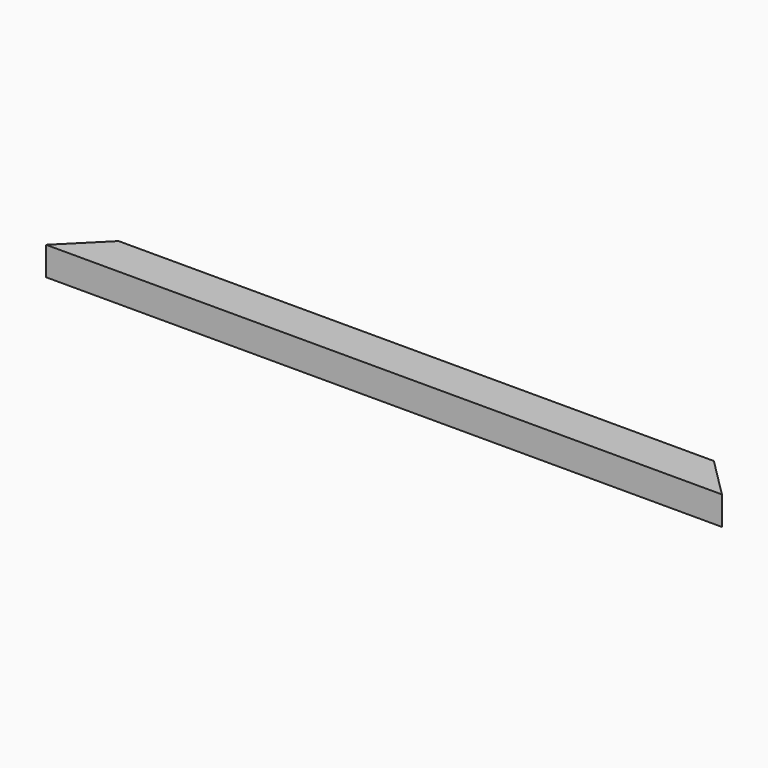
from build123d import *

# Parameters (mm, degrees)
F0_W       = 69
F0_H       = 49
F1_DEPTH   = 579
F2_T       = -4
F3_C1_SIZE = 68.9999
F3_C2_SIZE = 68.9999


# Not quite as in the source:
# - a fillet or chamfer is up to 0.001 mm smaller than in the source, because OpenCascade refuses the exact size


with BuildPart() as f1:
    # F0 (on Right) → F1 (new body, symmetric)
    with BuildSketch(Plane.YZ):
        Rectangle(F0_W, F0_H)
    extrude(amount=F1_DEPTH, both=True)

    # F2
    f2_openings = [f1.faces().sort_by_distance(p)[0] for p in [
        (579, 0, 0),
        (0, 34.5, 0),
        (-579, 0, 0),
    ]]
    offset(amount=F2_T, openings=f2_openings)

    # F3: chamfer of 69 on 4 edges, made by hand

    # F3_c1 (size 69 in the source; OpenCascade refuses exactly that, so slightly less here)
    f3_c1_edges = [f1.edges().sort_by_distance(p)[0] for p in [
        (579, 34.5, -22.5),
    ]]
    chamfer(f3_c1_edges, length=F3_C1_SIZE)

    # F3_c2 (size 69 in the source; OpenCascade refuses exactly that, so slightly less here)
    f3_c2_edges = [f1.edges().sort_by_distance(p)[0] for p in [
        (-579, 34.5, -22.5),
    ]]
    chamfer(f3_c2_edges, length=F3_C2_SIZE)


solid = f1.part
